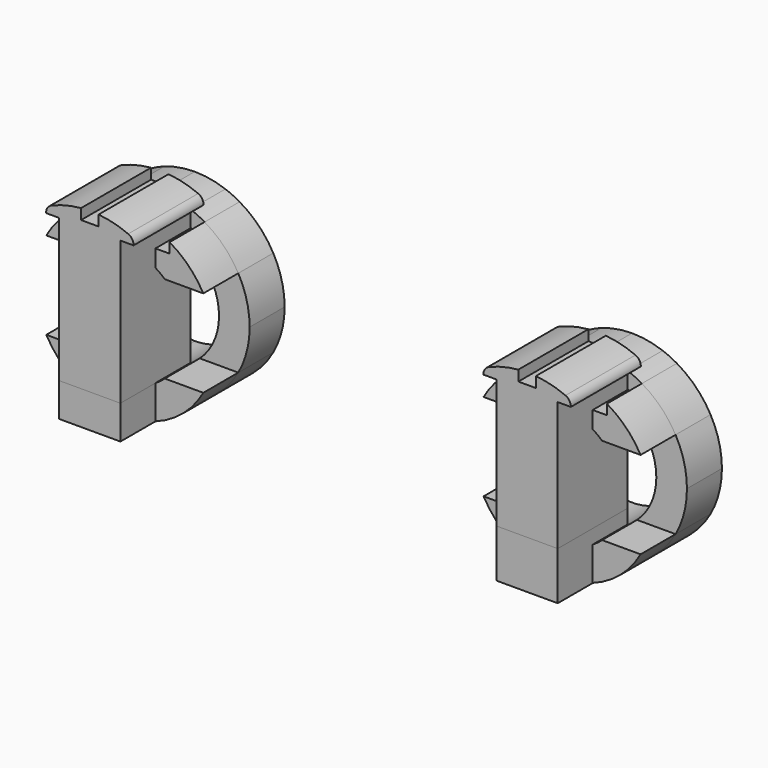
from build123d import *
from build123d import SkipClean  # not in build123d's __all__

# Parameters (mm, degrees)
F1_DEPTH = 1
F2_DEPTH = 1
F0_W     = 1.4
F0_H     = 0.37
F0_W_2   = 0.3
F0_H_2   = 2
F0_H_3   = 0.1601831752
F3_DEPTH = 2
F0_H_4   = 1.835
F0_H_5   = 0.165
F4_DEPTH = 2
F6_DEPTH = 3.001
F7_R     = 0.2
F7_2_R   = 0.2


# Not quite as in the source:
# - a feature names something its author has since deleted; it is built from what else it names


with BuildPart() as f1:
    # F0 (on Front) → F1 (new body)
    with BuildSketch(Plane.XZ):
        with BuildLine():
            ThreePointArc((-0.7, 1.9321037757), (-0.865797338, 1.8637113429), (-1.025, 1.7811232411))
            Line((-1.025, 1.7811232411), (-1.025, 1.55))
            Line((-1.025, 1.55), (-0.7, 1.55))
            Line((-0.7, 1.55), (-0.7, 1.9321037757))
        make_face()
        with BuildLine():
            Line((1.025, 1.55), (1.025, 1.7811232411))
            ThreePointArc((1.025, 1.7811232411), (0.865797338, 1.8637113429), (0.7, 1.9321037757))
            Line((0.7, 1.9321037757), (0.7, 1.55))
            Line((0.7, 1.55), (1.025, 1.55))
        make_face()
        with BuildLine():
            Line((0.9143440272, -1), (1.7952785299, -1))
            ThreePointArc((1.7952785299, -1), (1.9890101029, -0.5165886279), (2.055, 0))
            ThreePointArc((2.055, 0), (1.9890101029, 0.5165886279), (1.7952785299, 1))
            Line((1.7952785299, 1), (0.9143440272, 1))
            ThreePointArc((0.9143440272, 1), (1.2399518452, 0.5463921866), (1.355, 0))
            ThreePointArc((1.355, 0), (1.2399518452, -0.5463921866), (0.9143440272, -1))
        make_face()
        with BuildLine():
            ThreePointArc((-1.7952785299, 1), (-2.055, 0), (-1.7952785299, -1))
            Line((-1.7952785299, -1), (-0.9143440272, -1))
            ThreePointArc((-0.9143440272, -1), (-1.355, 0), (-0.9143440272, 1))
            Line((-0.9143440272, 1), (-1.7952785299, 1))
        make_face()
        with BuildLine():
            ThreePointArc((-1.7952785299, -1), (-1.3318438713, -1.5649974129), (-0.7, -1.9321037757))
            Line((-0.7, -1.9321037757), (-0.7, -1.355))
            Line((-0.7, -1.355), (-0.7, -1.1601831752))
            ThreePointArc((-0.7, -1.1601831752), (-0.8111358221, -1.0853956321), (-0.9143440272, -1))
            Line((-0.9143440272, -1), (-1.7952785299, -1))
        make_face()
        with BuildLine():
            Line((0.7, -1.355), (0.7, -1.9321037757))
            ThreePointArc((0.7, -1.9321037757), (1.3318438713, -1.5649974129), (1.7952785299, -1))
            Line((1.7952785299, -1), (0.9143440272, -1))
            ThreePointArc((0.9143440272, -1), (0.8111358221, -1.0853956321), (0.7, -1.1601831752))
            Line((0.7, -1.1601831752), (0.7, -1.355))
        make_face()
        with BuildLine():
            Line((0.7, -1.9321037757), (-0.7, -1.9321037757))
            ThreePointArc((-0.7, -1.9321037757), (0, -2.055), (0.7, -1.9321037757))
        make_face()
        with BuildLine():
            Line((0, -1.355), (0.7, -1.355))
            Line((0.7, -1.355), (0.7, -1.1601831752))
            ThreePointArc((0.7, -1.1601831752), (0.3633020765, -1.3053875291), (0, -1.355))
        make_face()
        with BuildLine():
            Line((-0.7, -1.1601831752), (-0.7, -1.355))
            Line((-0.7, -1.355), (0, -1.355))
            ThreePointArc((0, -1.355), (-0.3633020765, -1.3053875291), (-0.7, -1.1601831752))
        make_face()
        Polygon((-0.7, -1.355), (-0.7, -1.9321037757), (0.7, -1.9321037757), (0.7, -1.355), (0, -1.355), align=None)
        with BuildLine():
            ThreePointArc((0, 2.055), (-0.355353163, 2.0240427687), (-0.7, 1.9321037757))
            Line((-0.7, 1.9321037757), (-0.7, 1.55))
            Line((-0.7, 1.55), (0.7, 1.55))
            Line((0.7, 1.55), (0.7, 1.9321037757))
            ThreePointArc((0.7, 1.9321037757), (0.355353163, 2.0240427687), (0, 2.055))
        make_face()
        with BuildLine():
            Line((0.9143440272, 1), (1.7952785299, 1))
            ThreePointArc((1.7952785299, 1), (1.463226273, 1.442911596), (1.025, 1.7811232411))
            Line((1.025, 1.7811232411), (1.025, 1.55))
            Line((1.025, 1.55), (0.7, 1.55))
            Line((0.7, 1.55), (0.7, 1.1601831752))
            ThreePointArc((0.7, 1.1601831752), (0.8111358221, 1.0853956321), (0.9143440272, 1))
        make_face()
        with BuildLine():
            ThreePointArc((-1.025, 1.7811232411), (-1.463226273, 1.442911596), (-1.7952785299, 1))
            Line((-1.7952785299, 1), (-0.9143440272, 1))
            ThreePointArc((-0.9143440272, 1), (-0.8111358221, 1.0853956321), (-0.7, 1.1601831752))
            Line((-0.7, 1.1601831752), (-0.7, 1.55))
            Line((-0.7, 1.55), (-1.025, 1.55))
            Line((-1.025, 1.55), (-1.025, 1.7811232411))
        make_face()
        with BuildLine():
            Line((-0.7, 1.55), (-0.7, 1.1601831752))
            ThreePointArc((-0.7, 1.1601831752), (0, 1.355), (0.7, 1.1601831752))
            Line((0.7, 1.1601831752), (0.7, 1.55))
            Line((0.7, 1.55), (-0.7, 1.55))
        make_face()
    extrude(amount=-F1_DEPTH)

    # F0 (on Front) → F2, piece 2 (join)
    with BuildSketch(Plane.XZ):
        with BuildLine():
            ThreePointArc((-1.7952785299, -1), (-1.3318438713, -1.5649974129), (-0.7, -1.9321037757))
            Line((-0.7, -1.9321037757), (-0.7, -1.355))
            Line((-0.7, -1.355), (-0.7, -1.1601831752))
            ThreePointArc((-0.7, -1.1601831752), (-0.8111358221, -1.0853956321), (-0.9143440272, -1))
            Line((-0.9143440272, -1), (-1.7952785299, -1))
        make_face()
        with BuildLine():
            Line((0.7, -1.355), (0.7, -1.9321037757))
            ThreePointArc((0.7, -1.9321037757), (1.3318438713, -1.5649974129), (1.7952785299, -1))
            Line((1.7952785299, -1), (0.9143440272, -1))
            ThreePointArc((0.9143440272, -1), (0.8111358221, -1.0853956321), (0.7, -1.1601831752))
            Line((0.7, -1.1601831752), (0.7, -1.355))
        make_face()
        with BuildLine():
            ThreePointArc((-1.025, 1.7811232411), (-1.463226273, 1.442911596), (-1.7952785299, 1))
            Line((-1.7952785299, 1), (-0.9143440272, 1))
            ThreePointArc((-0.9143440272, 1), (-0.8111358221, 1.0853956321), (-0.7, 1.1601831752))
            Line((-0.7, 1.1601831752), (-0.7, 1.55))
            Line((-0.7, 1.55), (-1.025, 1.55))
            Line((-1.025, 1.55), (-1.025, 1.7811232411))
        make_face()
        with BuildLine():
            Line((0.9143440272, 1), (1.7952785299, 1))
            ThreePointArc((1.7952785299, 1), (1.463226273, 1.442911596), (1.025, 1.7811232411))
            Line((1.025, 1.7811232411), (1.025, 1.55))
            Line((1.025, 1.55), (0.7, 1.55))
            Line((0.7, 1.55), (0.7, 1.1601831752))
            ThreePointArc((0.7, 1.1601831752), (0.8111358221, 1.0853956321), (0.9143440272, 1))
        make_face()
    with SkipClean():  # cleaning this boolean's faces spoils the solid; the shape is the same uncleaned
        extrude(amount=F2_DEPTH)


with BuildPart() as f1b:
    # F0 (on Front) → F1, piece 2 (new body)
    with BuildSketch(Plane.XZ):
        with BuildLine():
            ThreePointArc((8.975, 1.7811232411), (8.536773727, 1.442911596), (8.2047214701, 1))
            Line((8.2047214701, 1), (9.0856559728, 1))
            ThreePointArc((9.0856559728, 1), (9.1888641779, 1.0853956321), (9.3, 1.1601831752))
            Line((9.3, 1.1601831752), (9.3, 1.55))
            Line((9.3, 1.55), (8.975, 1.55))
            Line((8.975, 1.55), (8.975, 1.7811232411))
        make_face()
        with BuildLine():
            Line((9.3, 1.55), (9.3, 1.1601831752))
            ThreePointArc((9.3, 1.1601831752), (10, 1.355), (10.7, 1.1601831752))
            Line((10.7, 1.1601831752), (10.7, 1.55))
            Line((10.7, 1.55), (9.3, 1.55))
        make_face()
        with BuildLine():
            ThreePointArc((10, 2.055), (9.644646837, 2.0240427687), (9.3, 1.9321037757))
            Line((9.3, 1.9321037757), (9.3, 1.55))
            Line((9.3, 1.55), (10.7, 1.55))
            Line((10.7, 1.55), (10.7, 1.9321037757))
            ThreePointArc((10.7, 1.9321037757), (10.355353163, 2.0240427687), (10, 2.055))
        make_face()
        with BuildLine():
            Line((10.7, 1.55), (10.7, 1.1601831752))
            ThreePointArc((10.7, 1.1601831752), (10.8111358221, 1.0853956321), (10.9143440272, 1))
            Line((10.9143440272, 1), (11.7952785299, 1))
            ThreePointArc((11.7952785299, 1), (11.463226273, 1.442911596), (11.025, 1.7811232411))
            Line((11.025, 1.7811232411), (11.025, 1.55))
            Line((11.025, 1.55), (10.7, 1.55))
        make_face()
        with BuildLine():
            Line((9.0856559728, -1), (8.2047214701, -1))
            ThreePointArc((8.2047214701, -1), (8.6681561287, -1.5649974129), (9.3, -1.9321037757))
            Line((9.3, -1.9321037757), (9.3, -1.1601831752))
            ThreePointArc((9.3, -1.1601831752), (9.1888641779, -1.0853956321), (9.0856559728, -1))
        make_face()
        with BuildLine():
            Line((9.3, -1.1601831752), (9.3, -1.9321037757))
            Line((9.3, -1.9321037757), (10.7, -1.9321037757))
            Line((10.7, -1.9321037757), (10.7, -1.1601831752))
            ThreePointArc((10.7, -1.1601831752), (10, -1.355), (9.3, -1.1601831752))
        make_face()
        with BuildLine():
            Line((10.7, -1.1601831752), (10.7, -1.9321037757))
            ThreePointArc((10.7, -1.9321037757), (11.3318438713, -1.5649974129), (11.7952785299, -1))
            Line((11.7952785299, -1), (10.9143440272, -1))
            ThreePointArc((10.9143440272, -1), (10.8111358221, -1.0853956321), (10.7, -1.1601831752))
        make_face()
        with BuildLine():
            Line((9.0856559728, 1), (8.2047214701, 1))
            ThreePointArc((8.2047214701, 1), (7.945, 0), (8.2047214701, -1))
            Line((8.2047214701, -1), (9.0856559728, -1))
            ThreePointArc((9.0856559728, -1), (8.645, 0), (9.0856559728, 1))
        make_face()
        with BuildLine():
            Line((10.6919537557, -1.935), (9.3080462443, -1.935))
            ThreePointArc((9.3080462443, -1.935), (10, -2.055), (10.6919537557, -1.935))
        make_face()
        with BuildLine():
            Line((10.9143440272, -1), (11.7952785299, -1))
            ThreePointArc((11.7952785299, -1), (11.9890101029, -0.5165886279), (12.055, 0))
            ThreePointArc((12.055, 0), (11.9890101029, 0.5165886279), (11.7952785299, 1))
            Line((11.7952785299, 1), (10.9143440272, 1))
            ThreePointArc((10.9143440272, 1), (11.2399518452, 0.5463921866), (11.355, 0))
            ThreePointArc((11.355, 0), (11.2399518452, -0.5463921866), (10.9143440272, -1))
        make_face()
        with BuildLine():
            Line((10.7, -1.9321037757), (9.3, -1.9321037757))
            ThreePointArc((9.3, -1.9321037757), (9.3040216156, -1.9335560733), (9.3080462443, -1.935))
            Line((9.3080462443, -1.935), (10.6919537557, -1.935))
            ThreePointArc((10.6919537557, -1.935), (10.6959783844, -1.9335560733), (10.7, -1.9321037757))
        make_face()
        with BuildLine():
            ThreePointArc((9.3, 1.9321037757), (9.134202662, 1.8637113429), (8.975, 1.7811232411))
            Line((8.975, 1.7811232411), (8.975, 1.55))
            Line((8.975, 1.55), (9.3, 1.55))
            Line((9.3, 1.55), (9.3, 1.9321037757))
        make_face()
        with BuildLine():
            Line((10.7, 1.9321037757), (10.7, 1.55))
            Line((10.7, 1.55), (11.025, 1.55))
            Line((11.025, 1.55), (11.025, 1.7811232411))
            ThreePointArc((11.025, 1.7811232411), (10.865797338, 1.8637113429), (10.7, 1.9321037757))
        make_face()
    extrude(amount=-F1_DEPTH)

    # F0 (on Front) → F2 (join)
    with BuildSketch(Plane.XZ):
        with BuildLine():
            ThreePointArc((8.975, 1.7811232411), (8.536773727, 1.442911596), (8.2047214701, 1))
            Line((8.2047214701, 1), (9.0856559728, 1))
            ThreePointArc((9.0856559728, 1), (9.1888641779, 1.0853956321), (9.3, 1.1601831752))
            Line((9.3, 1.1601831752), (9.3, 1.55))
            Line((9.3, 1.55), (8.975, 1.55))
            Line((8.975, 1.55), (8.975, 1.7811232411))
        make_face()
        with BuildLine():
            Line((10.7, 1.55), (10.7, 1.1601831752))
            ThreePointArc((10.7, 1.1601831752), (10.8111358221, 1.0853956321), (10.9143440272, 1))
            Line((10.9143440272, 1), (11.7952785299, 1))
            ThreePointArc((11.7952785299, 1), (11.463226273, 1.442911596), (11.025, 1.7811232411))
            Line((11.025, 1.7811232411), (11.025, 1.55))
            Line((11.025, 1.55), (10.7, 1.55))
        make_face()
        with BuildLine():
            Line((10.7, -1.1601831752), (10.7, -1.9321037757))
            ThreePointArc((10.7, -1.9321037757), (11.3318438713, -1.5649974129), (11.7952785299, -1))
            Line((11.7952785299, -1), (10.9143440272, -1))
            ThreePointArc((10.9143440272, -1), (10.8111358221, -1.0853956321), (10.7, -1.1601831752))
        make_face()
        with BuildLine():
            Line((9.0856559728, -1), (8.2047214701, -1))
            ThreePointArc((8.2047214701, -1), (8.6681561287, -1.5649974129), (9.3, -1.9321037757))
            Line((9.3, -1.9321037757), (9.3, -1.1601831752))
            ThreePointArc((9.3, -1.1601831752), (9.1888641779, -1.0853956321), (9.0856559728, -1))
        make_face()
    with SkipClean():  # cleaning this boolean's faces spoils the solid; the shape is the same uncleaned
        extrude(amount=F2_DEPTH)


with BuildPart() as f3:
    # F0 (on Front) → F3 (new body)
    with BuildSketch(Plane.XZ):
        with Locations((0, 2.3)):
            Rectangle(F0_W, F0_H)
        with Locations((-0.85, 2.3)):
            Rectangle(F0_W_2, F0_H)
        with Locations((0.85, 2.3)):
            Rectangle(F0_W_2, F0_H)
        with BuildLine():
            ThreePointArc((0, 2.055), (-0.355353163, 2.0240427687), (-0.7, 1.9321037757))
            Line((-0.7, 1.9321037757), (-0.7, 1.55))
            Line((-0.7, 1.55), (0.7, 1.55))
            Line((0.7, 1.55), (0.7, 1.9321037757))
            ThreePointArc((0.7, 1.9321037757), (0.355353163, 2.0240427687), (0, 2.055))
        make_face()
        with BuildLine():
            Line((0.7, 2.055), (0, 2.055))
            ThreePointArc((0, 2.055), (0.355353163, 2.0240427687), (0.7, 1.9321037757))
            Line((0.7, 1.9321037757), (0.7, 2.055))
        make_face()
        Polygon((-0.7, 2.055), (0, 2.055), (0.7, 2.055), (0.7, 2.115), (-0.7, 2.115), align=None)
        with BuildLine():
            Line((-0.7, 2.055), (-0.7, 1.9321037757))
            ThreePointArc((-0.7, 1.9321037757), (-0.355353163, 2.0240427687), (0, 2.055))
            Line((0, 2.055), (-0.7, 2.055))
        make_face()
        with BuildLine():
            Line((-0.7, 1.55), (-0.7, 1.1601831752))
            ThreePointArc((-0.7, 1.1601831752), (0, 1.355), (0.7, 1.1601831752))
            Line((0.7, 1.1601831752), (0.7, 1.55))
            Line((0.7, 1.55), (-0.7, 1.55))
        make_face()
        with BuildLine():
            Line((-0.7, 1.1601831752), (-0.7, 1))
            Line((-0.7, 1), (0.7, 1))
            Line((0.7, 1), (0.7, 1.1601831752))
            ThreePointArc((0.7, 1.1601831752), (0, 1.355), (-0.7, 1.1601831752))
        make_face()
        Rectangle(F0_W, F0_H_2)
        with Locations((0, -1.0800915876)):
            Rectangle(F0_W, F0_H_3)
    extrude(amount=F3_DEPTH)


with BuildPart() as f3b:
    # F0 (on Front) → F3, piece 2 (new body)
    with BuildSketch(Plane.XZ):
        with Locations((9.15, 2.3)):
            Rectangle(F0_W_2, F0_H)
        with Locations((10, 2.3)):
            Rectangle(F0_W, F0_H)
        with Locations((10.85, 2.3)):
            Rectangle(F0_W_2, F0_H)
        with BuildLine():
            ThreePointArc((10, 2.055), (9.644646837, 2.0240427687), (9.3, 1.9321037757))
            Line((9.3, 1.9321037757), (9.3, 1.55))
            Line((9.3, 1.55), (10.7, 1.55))
            Line((10.7, 1.55), (10.7, 1.9321037757))
            ThreePointArc((10.7, 1.9321037757), (10.355353163, 2.0240427687), (10, 2.055))
        make_face()
        with BuildLine():
            Line((9.3, 2.055), (9.3, 1.9321037757))
            ThreePointArc((9.3, 1.9321037757), (9.644646837, 2.0240427687), (10, 2.055))
            Line((10, 2.055), (9.3, 2.055))
        make_face()
        Polygon((9.3, 2.055), (10, 2.055), (10.7, 2.055), (10.7, 2.115), (9.3, 2.115), align=None)
        with BuildLine():
            Line((10.7, 2.055), (10, 2.055))
            ThreePointArc((10, 2.055), (10.355353163, 2.0240427687), (10.7, 1.9321037757))
            Line((10.7, 1.9321037757), (10.7, 2.055))
        make_face()
        with BuildLine():
            Line((9.3, 1.55), (9.3, 1.1601831752))
            ThreePointArc((9.3, 1.1601831752), (10, 1.355), (10.7, 1.1601831752))
            Line((10.7, 1.1601831752), (10.7, 1.55))
            Line((10.7, 1.55), (9.3, 1.55))
        make_face()
        with BuildLine():
            ThreePointArc((10.7, 1.1601831752), (10, 1.355), (9.3, 1.1601831752))
            Line((9.3, 1.1601831752), (9.3, 1))
            Line((9.3, 1), (10.7, 1))
            Line((10.7, 1), (10.7, 1.1601831752))
        make_face()
        with Locations((10, 0.0825)):
            Rectangle(F0_W, F0_H_4)
    extrude(amount=F3_DEPTH)


with BuildPart() as f4:
    # F0 (on Front) → F4 (new body)
    with BuildSketch(Plane.XZ):
        with Locations((10, -0.9175)):
            Rectangle(F0_W, F0_H_5)
        with BuildLine():
            Line((9.3, -1), (9.3, -1.1601831752))
            ThreePointArc((9.3, -1.1601831752), (10, -1.355), (10.7, -1.1601831752))
            Line((10.7, -1.1601831752), (10.7, -1))
            Line((10.7, -1), (9.3, -1))
        make_face()
        with BuildLine():
            Line((9.3, -1.1601831752), (9.3, -1.9321037757))
            Line((9.3, -1.9321037757), (10.7, -1.9321037757))
            Line((10.7, -1.9321037757), (10.7, -1.1601831752))
            ThreePointArc((10.7, -1.1601831752), (10, -1.355), (9.3, -1.1601831752))
        make_face()
        with BuildLine():
            ThreePointArc((9.3080462443, -1.935), (9.3040216156, -1.9335560733), (9.3, -1.9321037757))
            Line((9.3, -1.9321037757), (9.3, -1.935))
            Line((9.3, -1.935), (9.3080462443, -1.935))
        make_face()
        with BuildLine():
            Line((10.7, -1.9321037757), (9.3, -1.9321037757))
            ThreePointArc((9.3, -1.9321037757), (9.3040216156, -1.9335560733), (9.3080462443, -1.935))
            Line((9.3080462443, -1.935), (10.6919537557, -1.935))
            ThreePointArc((10.6919537557, -1.935), (10.6959783844, -1.9335560733), (10.7, -1.9321037757))
        make_face()
        with BuildLine():
            Line((10.7, -1.935), (10.7, -1.9321037757))
            ThreePointArc((10.7, -1.9321037757), (10.6959783844, -1.9335560733), (10.6919537557, -1.935))
            Line((10.6919537557, -1.935), (10.7, -1.935))
        make_face()
    extrude(amount=F4_DEPTH)


with BuildPart() as f4b:
    # F0 (on Front) → F4, piece 2 (new body)
    with BuildSketch(Plane.XZ):
        with BuildLine():
            Line((0.7, -1.1601831752), (-0.7, -1.1601831752))
            ThreePointArc((-0.7, -1.1601831752), (-0.3633020765, -1.3053875291), (0, -1.355))
            ThreePointArc((0, -1.355), (0.3633020765, -1.3053875291), (0.7, -1.1601831752))
        make_face()
        with BuildLine():
            Line((-0.7, -1.1601831752), (-0.7, -1.355))
            Line((-0.7, -1.355), (0, -1.355))
            ThreePointArc((0, -1.355), (-0.3633020765, -1.3053875291), (-0.7, -1.1601831752))
        make_face()
        with BuildLine():
            Line((0, -1.355), (0.7, -1.355))
            Line((0.7, -1.355), (0.7, -1.1601831752))
            ThreePointArc((0.7, -1.1601831752), (0.3633020765, -1.3053875291), (0, -1.355))
        make_face()
        Polygon((-0.7, -1.355), (-0.7, -1.9321037757), (0.7, -1.9321037757), (0.7, -1.355), (0, -1.355), align=None)
    extrude(amount=F4_DEPTH)


with BuildPart() as f6_tool:
    # F5 (on face) → F6 (new body, through all)
    with BuildSketch(Plane.XZ.offset(2)):
        with BuildLine():
            ThreePointArc((0.2, 2.4760934831), (0.7525867121, 2.3554040277), (1.2576146983, 2.1007184329))
            Line((1.2576146983, 2.1007184329), (1.2576146983, 2.9572506901))
            Line((1.2576146983, 2.9572506901), (-1.2576146983, 2.9572506901))
            Line((-1.2576146983, 2.9572506901), (-1.2576146983, 2.1007184329))
            ThreePointArc((-1.2576146983, 2.1007184329), (-0.7525867121, 2.3554040277), (-0.2, 2.4760934831))
            Line((-0.2, 2.4760934831), (-0.2, 2.735))
            Line((-0.2, 2.735), (0.2, 2.735))
            Line((0.2, 2.735), (0.2, 2.4760934831))
        make_face()
        with BuildLine():
            Line((0.2, 2.235), (0.2, 2.4760934831))
            ThreePointArc((0.2, 2.4760934831), (0, 2.485), (-0.2, 2.4760934831))
            Line((-0.2, 2.4760934831), (-0.2, 2.235))
            Line((-0.2, 2.235), (0.2, 2.235))
        make_face()
        with BuildLine():
            ThreePointArc((-0.2, 2.4760934831), (0, 2.485), (0.2, 2.4760934831))
            Line((0.2, 2.4760934831), (0.2, 2.735))
            Line((0.2, 2.735), (-0.2, 2.735))
            Line((-0.2, 2.735), (-0.2, 2.4760934831))
        make_face()
        with BuildLine():
            ThreePointArc((10.2, 2.4760934831), (10.6105045763, 2.4005909499), (11, 2.2505644371))
            Line((11, 2.2505644371), (11, 2.485))
            Line((11, 2.485), (10.2, 2.485))
            Line((10.2, 2.485), (10.2, 2.4760934831))
        make_face()
        with BuildLine():
            Line((9, 2.485), (9, 2.2505644371))
            ThreePointArc((9, 2.2505644371), (9.3894954237, 2.4005909499), (9.8, 2.4760934831))
            Line((9.8, 2.4760934831), (9.8, 2.485))
            Line((9.8, 2.485), (9, 2.485))
        make_face()
        with BuildLine():
            Line((10.2, 2.235), (10.2, 2.4760934831))
            ThreePointArc((10.2, 2.4760934831), (10.1000991084, 2.4827722679), (10, 2.485))
            ThreePointArc((10, 2.485), (9.8999008916, 2.4827722679), (9.8, 2.4760934831))
            Line((9.8, 2.4760934831), (9.8, 2.235))
            Line((9.8, 2.235), (10.2, 2.235))
        make_face()
        with BuildLine():
            ThreePointArc((10, 2.485), (10.1000991084, 2.4827722679), (10.2, 2.4760934831))
            Line((10.2, 2.4760934831), (10.2, 2.485))
            Line((10.2, 2.485), (10, 2.485))
        make_face()
        with BuildLine():
            Line((9.8, 2.485), (9.8, 2.4760934831))
            ThreePointArc((9.8, 2.4760934831), (9.8999008916, 2.4827722679), (10, 2.485))
            Line((10, 2.485), (9.8, 2.485))
        make_face()
        Polygon((9.8, 2.485), (10, 2.485), (10.2, 2.485), (10.2, 2.735), (9.8, 2.735), align=None)
    extrude(amount=-F6_DEPTH)


with BuildPart() as f3_1:
    add(f3.part, clean=False)

    # F6: cut by f6_tool
    add(f6_tool.part, mode=Mode.SUBTRACT)

    # F7
    f7_edges = [f3_1.edges().sort_by_distance(p)[0] for p in [
        (-1, -1, 2.250564),
        (1, -1, 2.250564),
    ]]
    fillet(f7_edges, radius=F7_R)


with BuildPart() as f3b_1:
    add(f3b.part, clean=False)

    # F6: cut by f6_tool
    add(f6_tool.part, mode=Mode.SUBTRACT)

    # F7#2
    f7_2_edges = [f3b_1.edges().sort_by_distance(p)[0] for p in [
        (11, -1, 2.250564),
        (9, -1, 2.250564),
    ]]
    fillet(f7_2_edges, radius=F7_2_R)


solid = Compound([f1.part, f1b.part, f4.part, f4b.part, f3_1.part, f3b_1.part])
